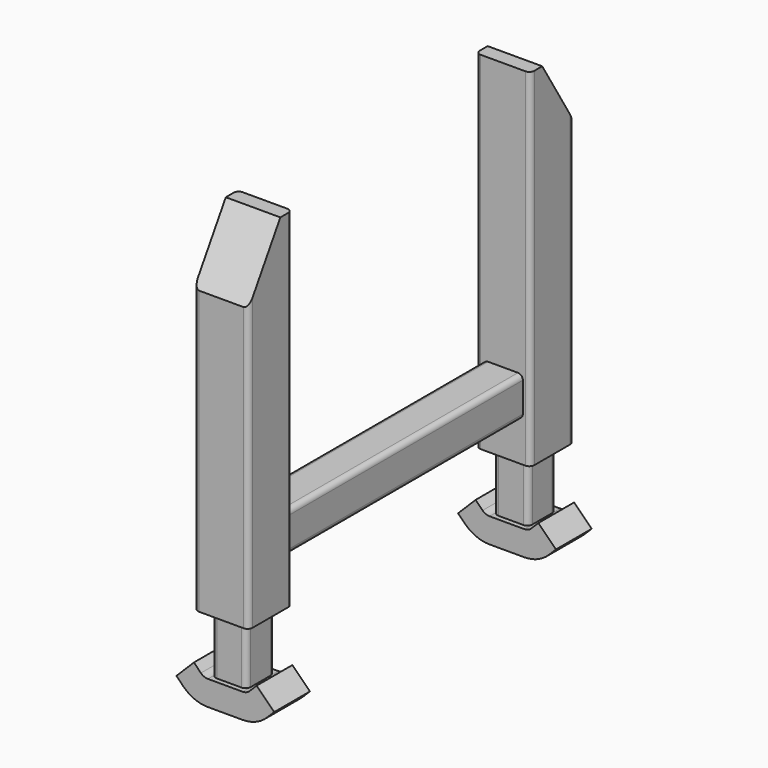
from build123d import *

# Parameters (mm, degrees)
F0_W         = 1.1
F0_H         = 7
F1_DEPTH     = 0.55
F2_W         = 0.7
F2_H         = 0.7
F3_DEPTH     = 1.2
F4_R         = 0.1
F7_DEPTH     = 0.45
F8_W         = 0.8
F8_H         = 0.8
F9_DEPTH     = 3
F10_R        = 0.1
F11_T1_DEPTH = 7.6228122918


# Not quite as in the source:
# - a fillet or chamfer that OpenCascade refuses, or shapes differently, is made with other operations: its cross-section is extruded or revolved along the edge and cut away or added


with BuildPart() as f1:
    # F0 (on Right) → F1 (new body, symmetric)
    with BuildSketch(Plane.YZ):
        with Locations((3.55, -3.5)):
            Rectangle(F0_W, F0_H)
    extrude(amount=F1_DEPTH, both=True)

    # F2 (on face) → F3 (join)
    with BuildSketch(Plane(origin=(0, 0, -7), x_dir=(1, 0, 0), z_dir=(0, 0, -1))):
        with Locations((0, -3.55)):
            Rectangle(F2_W, F2_H)
    extrude(amount=F3_DEPTH)

    # F4
    f4_edges = [f1.edges().sort_by_distance(p)[0] for p in [
        (0.55, 4.1, -3.5),
        (0.55, 3, -3.5),
        (-0.55, 4.1, -3.5),
        (0.35, 3.9, -7.6),
        (-0.35, 3.9, -7.6),
        (0.35, 3.2, -7.6),
        (-0.35, 3.2, -7.6),
        (-0.55, 3, -3.5),
    ]]
    fillet(f4_edges, radius=F4_R)

    # F6 (on mid) → F7 (join, symmetric)
    with BuildSketch(Plane(origin=(0, 3.55, 0), x_dir=(-1, 0, 0), z_dir=(0, 1, 0))):
        with BuildLine():
            ThreePointArc((0.4914213562, -8.1414213562), (0.4265366865, -8.1847759065), (0.35, -8.2))
            Line((0.35, -8.2), (-0.35, -8.2))
            ThreePointArc((-0.35, -8.2), (-0.4265366865, -8.1847759065), (-0.4914213562, -8.1414213562))
            Line((-0.4914213562, -8.1414213562), (-0.6328427125, -8))
            Line((-0.6328427125, -8), (-0.9863961031, -8.3535533906))
            Line((-0.9863961031, -8.3535533906), (-0.8449747468, -8.4949747468))
            ThreePointArc((-0.8449747468, -8.4949747468), (-0.6178784027, -8.6467156728), (-0.35, -8.7))
            Line((-0.35, -8.7), (0.35, -8.7))
            ThreePointArc((0.35, -8.7), (0.6178784027, -8.6467156728), (0.8449747468, -8.4949747468))
            Line((0.8449747468, -8.4949747468), (0.9863961031, -8.3535533906))
            Line((0.9863961031, -8.3535533906), (0.6328427125, -8))
            Line((0.6328427125, -8), (0.4914213562, -8.1414213562))
        make_face()
    extrude(amount=F7_DEPTH, both=True)

    # F8 (on face) → F9 (join, through all)
    with BuildSketch(Plane.XZ.offset(-3)):
        with Locations((0, -5.8)):
            Rectangle(F8_W, F8_H)
    extrude(amount=F9_DEPTH)

    # F10
    f10_edges = [f1.edges().sort_by_distance(p)[0] for p in [
        (-0.4, 1.5, -5.4),
        (-0.4, 1.5, -6.2),
        (0.4, 1.5, -6.2),
        (0.4, 1.5, -5.4),
    ]]
    fillet(f10_edges, radius=F10_R)

    # F11: chamfer of 0.8 x 1.3 on 1 edges, made by hand

    # F11_s2 → F11_t1 (cut)
    with BuildSketch(Plane.YZ.offset(-3.8114061459)):
        Polygon((3.3, 0), (4.1, -1.3), (4.1, 0), align=None)
    extrude(amount=F11_T1_DEPTH, mode=Mode.SUBTRACT)

    # F12: F1 across plane


with BuildPart() as f1_1:
    add(f1.part)
    add(f1.part.mirror(Plane.XZ))


solid = f1_1.part
